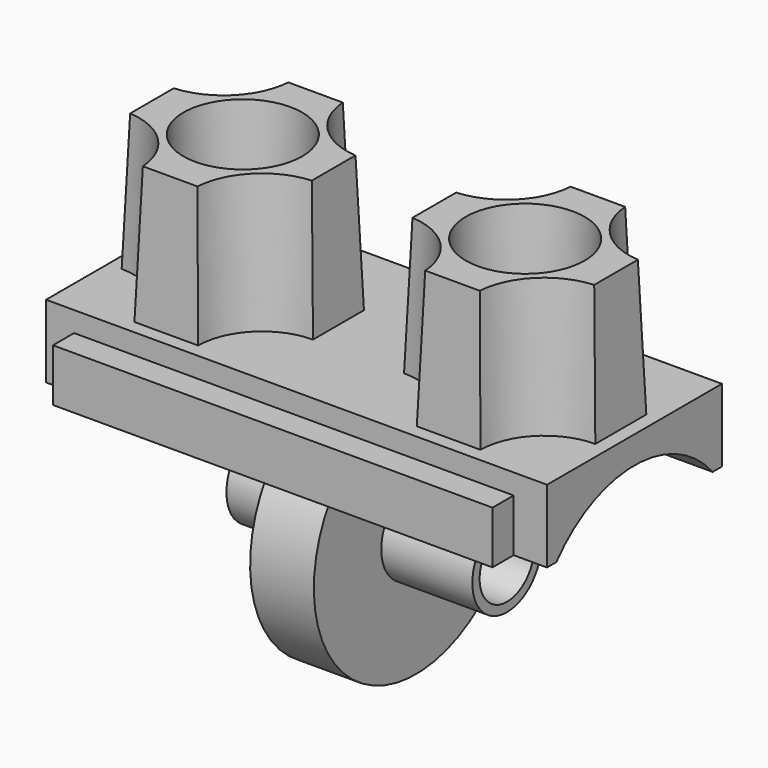
from build123d import *

# Parameters (mm, degrees)
F0_W                    = 55
F0_H                    = 24
F1_DEPTH                = 8
F2_R                    = 14
F3_DEPTH                = 63.70195
F4_R                    = 14
F5_DEPTH                = 3.5
F5_DEPTH_BACK           = 3.5
F6_R                    = 4.75
F6_R_2                  = 3.75
F7_DEPTH                = 10
F9_R                    = 6
F10_DEPTH               = 15
DRAFT_F10_DRAFTED_ANGLE = 2
F13_START               = 11.1
F12_W                   = 48.2565797865
F12_H                   = 5.7730269618
F13_DEPTH               = 3.8


# Not quite as in the source:
# - an extrude with a draft is written as a straight extrude whose walls are then drafted


with BuildPart() as f1:
    # F0 (on Top) → F1 (new body)
    with BuildSketch(Plane.XY):
        Rectangle(F0_W, F0_H)
    extrude(amount=F1_DEPTH)

    # F2 (on face) → F3 (cut)
    with BuildSketch(Plane(origin=(-27.5, 0, 0), x_dir=(0, -1, 0), z_dir=(-1, 0, 0))):
        with Locations((0, -9)):
            Circle(F2_R)
    extrude(amount=-F3_DEPTH, mode=Mode.SUBTRACT)

    # F4 (on Right) → F5 (join, two sides)
    with BuildSketch(Plane.YZ) as f5_sk:
        with Locations((0, -9)):
            Circle(F4_R)
    extrude(amount=F5_DEPTH)
    extrude(f5_sk.sketch, amount=-F5_DEPTH_BACK)

    # F6 (on face) → F7 (join)
    with BuildSketch(Plane.YZ.offset(3.5)):
        with Locations((0, -9)):
            Circle(F6_R)
        with Locations((0, -9)):
            Circle(F6_R_2, mode=Mode.SUBTRACT)
    extrude(amount=F7_DEPTH)

    # F8: F1 across plane


with BuildPart() as f1_1:
    add(f1.part)
    add(f1.part.mirror(Plane.YZ))


with BuildPart() as f10_drafted:
    # F9 (on face) → F10 (new body)
    with BuildSketch(Plane.XY.offset(8)):
        with BuildLine():
            Line((-12, 10.5), (-19, 10.5))
            ThreePointArc((-19, 10.5), (-21.0502525317, 5.5502525317), (-26, 3.5))
            Line((-26, 3.5), (-26, -3.5))
            ThreePointArc((-26, -3.5), (-21.0502525317, -5.5502525317), (-19, -10.5))
            Line((-19, -10.5), (-12, -10.5))
            ThreePointArc((-12, -10.5), (-9.9497474683, -5.5502525317), (-5, -3.5))
            Line((-5, -3.5), (-5, 3.5))
            ThreePointArc((-5, 3.5), (-9.9497474683, 5.5502525317), (-12, 10.5))
        make_face()
        with Locations((-15.5, 0)):
            Circle(F9_R, mode=Mode.SUBTRACT)
    extrude(amount=F10_DEPTH)

    # draft_F10_drafted
    draft_f10_drafted_walls = [f10_drafted.faces().sort_by_distance(p)[0] for p in [
        (-9.9497474683, 5.5502525317, 18),
        (-15.5, 10.5, 18),
        (-21.0502525317, 5.5502525317, 18),
        (-26, 0, 18),
        (-21.0502525317, -5.5502525317, 18),
        (-15.5, -10.5, 18),
        (-9.9497474683, -5.5502525317, 18),
        (-5, 0, 18),
        (-21.5, 0, 18),
    ]]
    draft(draft_f10_drafted_walls, neutral_plane=Plane.XY.offset(8), angle=DRAFT_F10_DRAFTED_ANGLE)


with BuildPart() as f1_2:
    add(f1_1.part)

    # join_F10_drafted: union F10_drafted
    add(f10_drafted.part)

    # F11: F1 across plane


with BuildPart() as f1_3:
    add(f1_2.part)
    add(f1_2.part.mirror(Plane.YZ))

    # F12 (on Front) → F13 (join)
    with BuildSketch(Plane.XZ.offset(F13_START)):
        with Locations((-0.2960525453, 2.8865134809)):
            Rectangle(F12_W, F12_H)
    extrude(amount=F13_DEPTH)


solid = f1_3.part
